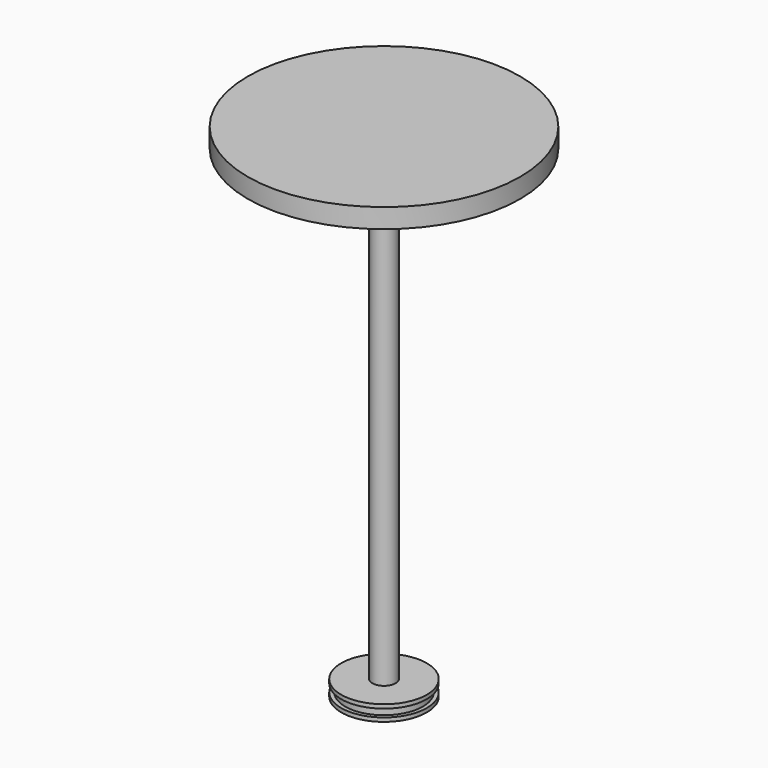
from build123d import *

# Parameters (mm, degrees)
F0_R     = 175
F1_DEPTH = 25
F2_R     = 15
F3_DEPTH = 600
F4_R     = 55
F4_R_2   = 15
F5_DEPTH = 5
F6_R     = 50
F7_DEPTH = 10
F8_R     = 55
F8_R_2   = 50
F9_DEPTH = 5


with BuildPart() as f1:
    # F0 (on Top) → F1 (new body)
    with BuildSketch(Plane.XY):
        Circle(F0_R)
    extrude(amount=F1_DEPTH)

    # F2 (on face) → F3 (join)
    with BuildSketch(Plane(origin=(0, 0, 0), x_dir=(1, 0, 0), z_dir=(0, 0, -1))):
        Circle(F2_R)
    extrude(amount=F3_DEPTH)

    # F4 (on face) → F5 (join)
    with BuildSketch(Plane(origin=(0, 0, -600), x_dir=(1, 0, 0), z_dir=(0, 0, -1))):
        Circle(F4_R)
        Circle(F4_R_2, mode=Mode.SUBTRACT)
        Circle(F4_R_2)
    extrude(amount=F5_DEPTH)

    # F6 (on face) → F7 (join)
    with BuildSketch(Plane(origin=(0, 0, -605), x_dir=(1, 0, 0), z_dir=(0, 0, -1))):
        Circle(F6_R)
    extrude(amount=F7_DEPTH)

    # F8 (on face) → F9 (join)
    with BuildSketch(Plane(origin=(0, 0, -615), x_dir=(1, 0, 0), z_dir=(0, 0, -1))):
        Circle(F8_R)
        Circle(F8_R_2, mode=Mode.SUBTRACT)
        Circle(F8_R_2)
    extrude(amount=F9_DEPTH)


solid = f1.part
